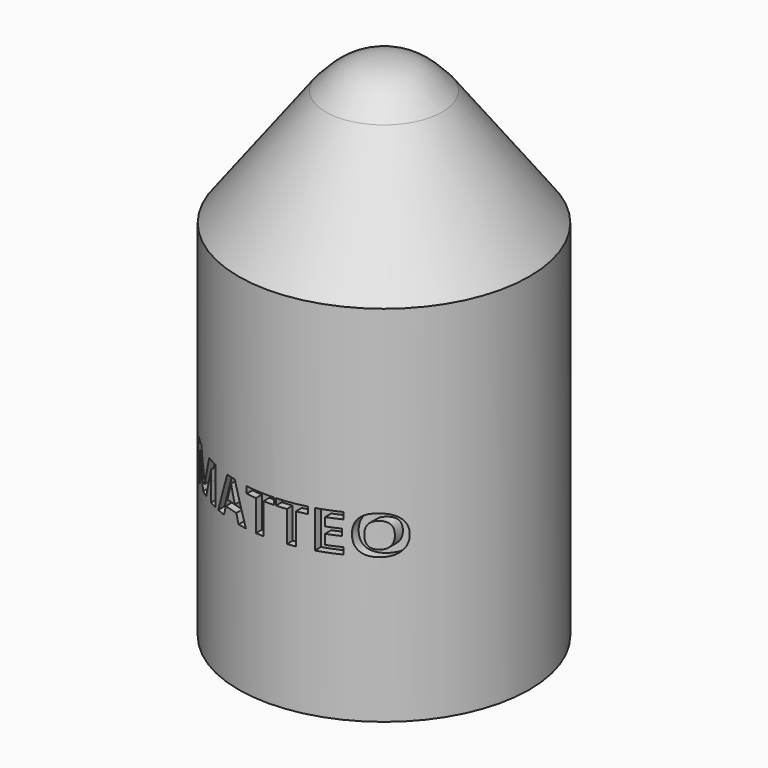
from build123d import *

# Parameters (mm, degrees)
F0_R         = 20
F0_R_2       = 19
F1_DEPTH     = 50
F4_TEXT_SIZE = 7.2226610992
F5_DEPTH     = 53.89573


# Not quite as in the source:
# - Text() gives the source's letters only with a copy of the font that has no kerning and outlines rounded to 1/6400 em; it was checked with that copy


with BuildPart() as f1:
    # F0 (on Top) → F1 (new body)
    with BuildSketch(Plane.XY):
        Circle(F0_R)
        Circle(F0_R_2, mode=Mode.SUBTRACT)
    extrude(amount=F1_DEPTH)

    # F2 (on Front) → F3 (revolve)
    with BuildSketch(Plane.XZ):
        with BuildLine():
            Line((0, 70), (0, 50))
            Line((0, 50), (20, 50))
            Line((20, 50), (8, 66))
            add(Edge.make_bspline(
                [(8, 66), (5.3391167894, 69.0013170242), (3.4907322843, 70.0460597873), (0, 70)],
                knots=[0, 0, 0, 0, 8.94427191, 8.94427191, 8.94427191, 8.94427191], degree=3))
        make_face()
    revolve(axis=Axis((0, 0, 60), (0, 0, 1)))

    # F4 (on Front) → F5 (cut)
    with BuildSketch(Plane.XZ):
        with Locations((-15, 20)):
            Text('MATTEO', F4_TEXT_SIZE, font='Open Sans', font_style=FontStyle.BOLD, text_align=(TextAlign.LEFT, TextAlign.BOTTOM))
    extrude(amount=F5_DEPTH, mode=Mode.SUBTRACT)


solid = f1.part
